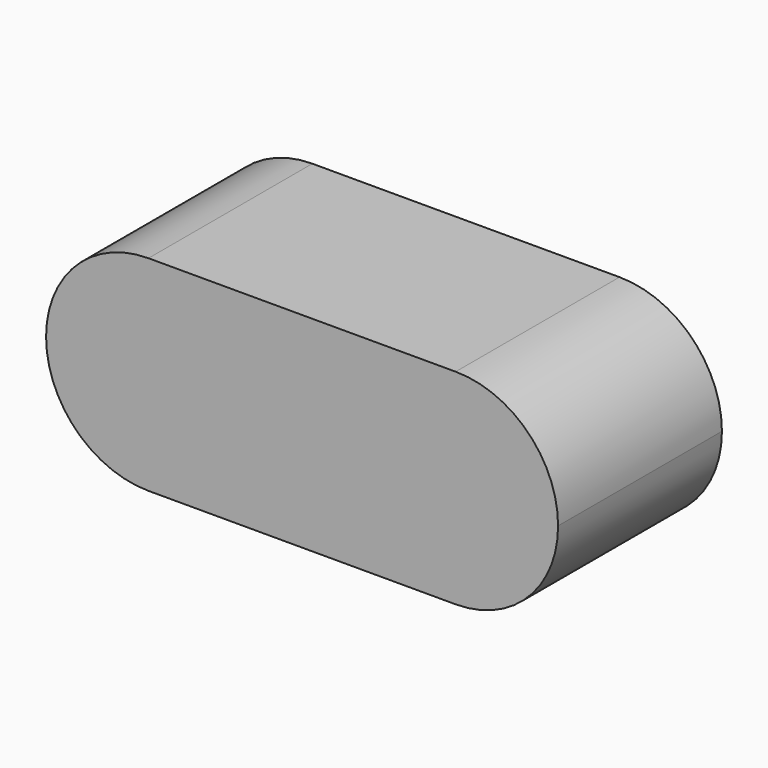
from build123d import *

# Parameters (mm, degrees)
F0_W     = 50
F0_H     = 20
F1_DEPTH = 20
F2_R     = 9.99999


# Not quite as in the source:
# - a fillet or chamfer is up to 0.001 mm smaller than in the source, because OpenCascade refuses the exact size


with BuildPart() as f1:
    # F0 (on Top) → F1 (new body)
    with BuildSketch(Plane.XY):
        with Locations((-25, 10)):
            Rectangle(F0_W, F0_H)
    extrude(amount=F1_DEPTH)

    # F2 (radius 10 in the source; OpenCascade refuses exactly that, so slightly less here)
    f2_edges = [f1.edges().sort_by_distance(p)[0] for p in [
        (-50, 10, 20),
        (0, 10, 20),
        (0, 10, 0),
        (-50, 10, 0),
    ]]
    fillet(f2_edges, radius=F2_R)


solid = f1.part
